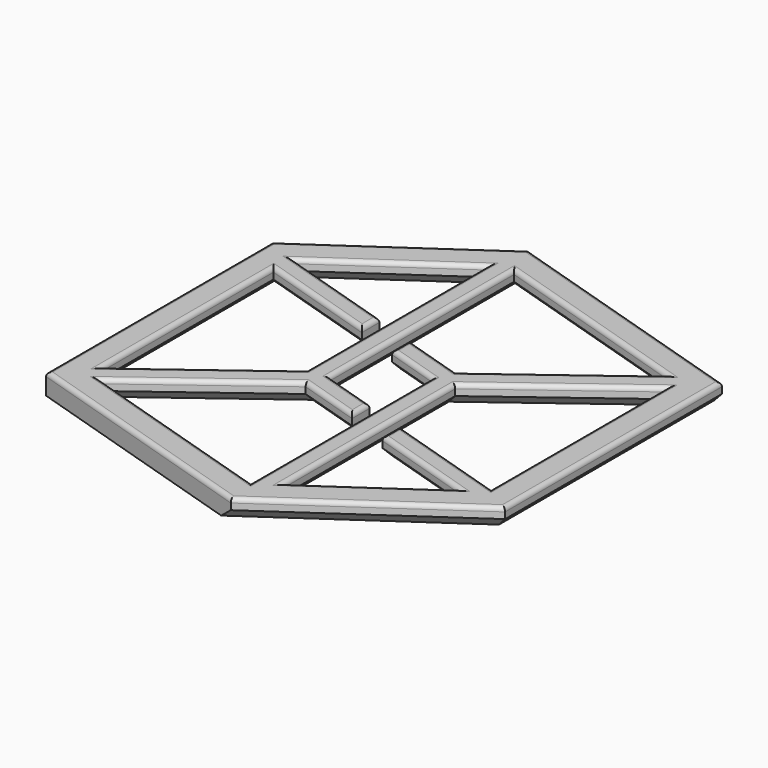
from build123d import *

# Parameters (mm, degrees)
F1_DEPTH = 2
F2_SIZE  = 0.99999
F3_R     = 0.4


# Not quite as in the source:
# - a fillet or chamfer is up to 0.001 mm smaller than in the source, because OpenCascade refuses the exact size
# - a feature names something its author has since deleted; it is built from what else it names


with BuildPart() as f1:
    # F0 (on Top) → F1 (new body)
    with BuildSketch(Plane.XY):
        Polygon((-13.8196714956, 16.8550248196), (-29.5628140081, 5.986613122), (-29.5628140081, -20.895469086), (-6.1378714726, -28.2046662626), (10.6815792442, -16.5932160853), (10.6815792442, 9.2099912209), align=None)
        Polygon((-5.5893215574, -24.5450593134), (-6.5893215574, -25.2354177783), (-25.6853743411, -19.2769478747), (-26.8628140101, -18.9095557801), (-26.8628140101, -17.6600457129), (-26.8628140101, 2.7856210558), (-26.8628140101, 4.569670104), (-26.5525036512, 4.783895487), (-14.6640113722, 12.9912167666), (-13.6640113722, 13.6815752315), (-13.3682214107, 13.8857763353), (-12.6640113722, 13.6660443117), (6.8041395773, 7.5914700096), (7.9815792463, 7.224077915), (7.9815792463, 5.9745678478), (7.9815792463, -14.864596124), (7.9815792463, -15.1762730673), (7.5702731242, -15.4602217303), (6.2023996294, -16.4045447763), (-4.5893215574, -23.8547008485), align=None, mode=Mode.SUBTRACT)
        Polygon((-26.8628140101, 4.569670104), (-26.8628140101, 2.7856210558), (-15.6640113722, -0.7086994318), (-15.6640113722, 1.3863999797), (-26.5525036512, 4.783895487), align=None)
        with BuildLine():
            Line((-13.6640113722, 13.6815752315), (-13.6640113722, -8.0212351043))
            ThreePointArc((-13.6640113722, -8.0212351043), (-13.5133605177, -8.0326480722), (-13.3661484098, -8.0666264642))
            Line((-13.3661484098, -8.0666264642), (-12.6640113722, -8.2857116571))
            Line((-12.6640113722, -8.2857116571), (-12.6640113722, 13.6660443117))
            Line((-12.6640113722, 13.6660443117), (-13.3682214107, 13.8857763353))
            Line((-13.3682214107, 13.8857763353), (-13.6640113722, 13.6815752315))
        make_face()
        with BuildLine():
            Line((-14.6640113722, 12.9912167666), (-14.6640113722, -8.5209081976))
            Line((-14.6640113722, -8.5209081976), (-14.2635929044, -8.2209214243))
            ThreePointArc((-14.2635929044, -8.2209214243), (-13.9799910551, -8.0724691479), (-13.6640113722, -8.0212351043))
            Line((-13.6640113722, -8.0212351043), (-13.6640113722, 13.6815752315))
            Line((-13.6640113722, 13.6815752315), (-14.6640113722, 12.9912167666))
        make_face()
        with BuildLine():
            Line((-6.5893215574, -3.6785358878), (-6.5893215574, -25.2354177783))
            Line((-6.5893215574, -25.2354177783), (-5.5893215574, -24.5450593134))
            Line((-5.5893215574, -24.5450593134), (-5.5893215574, -3.9430124406))
            ThreePointArc((-5.5893215574, -3.9430124406), (-5.739972412, -3.9315994727), (-5.8871845198, -3.8976210807))
            Line((-5.8871845198, -3.8976210807), (-6.5893215574, -3.6785358878))
        make_face()
        with BuildLine():
            Line((-5.5893215574, -3.9430124406), (-5.5893215574, -24.5450593134))
            Line((-5.5893215574, -24.5450593134), (-4.5893215574, -23.8547008485))
            Line((-4.5893215574, -23.8547008485), (-4.5893215574, -3.4433393473))
            Line((-4.5893215574, -3.4433393473), (-4.9897400253, -3.7433261206))
            ThreePointArc((-4.9897400253, -3.7433261206), (-5.2733418745, -3.891778397), (-5.5893215574, -3.9430124406))
        make_face()
        with BuildLine():
            ThreePointArc((-5.2914585951, -1.9884038006), (-5.0122521974, -2.1263172994), (-4.7890078775, -2.3434309085))
            Line((-4.7890078775, -2.3434309085), (7.9815792463, 7.224077915))
            Line((7.9815792463, 7.224077915), (6.8041395773, 7.5914700096))
            Line((6.8041395773, 7.5914700096), (-5.7796330622, -1.8360805481))
            Line((-5.7796330622, -1.8360805481), (-5.2914585951, -1.9884038006))
        make_face()
        with BuildLine():
            Line((-4.5893215574, -2.9430124406), (-4.5893215574, -3.4433393473))
            Line((-4.5893215574, -3.4433393473), (7.9815792463, 5.9745678478))
            Line((7.9815792463, 5.9745678478), (7.9815792463, 7.224077915))
            Line((7.9815792463, 7.224077915), (-4.7890078775, -2.3434309085))
            ThreePointArc((-4.7890078775, -2.3434309085), (-4.6405556011, -2.6270327577), (-4.5893215574, -2.9430124406))
        make_face()
        with BuildLine():
            Line((-26.8628140101, -18.9095557801), (-25.6853743411, -19.2769478747))
            Line((-25.6853743411, -19.2769478747), (-13.4736998674, -10.1281669968))
            Line((-13.4736998674, -10.1281669968), (-13.9618743346, -9.9758437443))
            ThreePointArc((-13.9618743346, -9.9758437443), (-14.2410807322, -9.8379302455), (-14.4643250521, -9.6208166364))
            Line((-14.4643250521, -9.6208166364), (-26.8628140101, -18.9095557801))
        make_face()
        with BuildLine():
            Line((-26.8628140101, -17.6600457129), (-26.8628140101, -18.9095557801))
            Line((-26.8628140101, -18.9095557801), (-14.4643250521, -9.6208166364))
            ThreePointArc((-14.4643250521, -9.6208166364), (-14.6127773286, -9.3372147872), (-14.6640113722, -9.0212351043))
            Line((-14.6640113722, -9.0212351043), (-14.6640113722, -8.5209081976))
            Line((-14.6640113722, -8.5209081976), (-26.8628140101, -17.6600457129))
        make_face()
        Polygon((-3.5893215574, -13.3492706494), (6.2023996294, -16.4045447763), (7.5702731242, -15.4602217303), (-3.5893215574, -11.9781351546), align=None)
        with BuildLine():
            Line((-11.6640113722, -2.0950994115), (-6.5893215574, -3.6785358878))
            Line((-6.5893215574, -3.6785358878), (-6.5893215574, -2.9430124406))
            ThreePointArc((-6.5893215574, -2.9430124406), (-6.4836317755, -2.4955649757), (-6.1889030896, -2.1426987607))
            Line((-6.1889030896, -2.1426987607), (-5.7796330622, -1.8360805481))
            Line((-5.7796330622, -1.8360805481), (-11.6640113722, 0))
            Line((-11.6640113722, 0), (-11.6640113722, -2.0950994115))
        make_face()
        with BuildLine():
            Line((-13.06442984, -9.8215487842), (-13.4736998674, -10.1281669968))
            Line((-13.4736998674, -10.1281669968), (-7.5893215574, -11.9642475449))
            Line((-7.5893215574, -11.9642475449), (-7.5893215574, -9.8691481334))
            Line((-7.5893215574, -9.8691481334), (-12.6640113722, -8.2857116571))
            Line((-12.6640113722, -8.2857116571), (-12.6640113722, -9.0212351043))
            ThreePointArc((-12.6640113722, -9.0212351043), (-12.7697011542, -9.4686825693), (-13.06442984, -9.8215487842))
        make_face()
        Polygon((-3.5893215574, -11.9781351546), (7.5702731242, -15.4602217303), (7.9815792463, -15.1762730673), (7.9815792463, -14.864596124), (-3.5893215574, -11.2541712379), align=None)
        with BuildLine():
            ThreePointArc((-5.8871845198, -3.8976210807), (-5.739972412, -3.9315994727), (-5.5893215574, -3.9430124406))
            Line((-5.5893215574, -3.9430124406), (-5.5893215574, -2.9430124406))
            Line((-5.5893215574, -2.9430124406), (-4.7890078775, -2.3434309085))
            ThreePointArc((-4.7890078775, -2.3434309085), (-5.0122521974, -2.1263172994), (-5.2914585951, -1.9884038006))
            ThreePointArc((-5.2914585951, -1.9884038006), (-5.7587625723, -1.9574721104), (-6.1889030896, -2.1426987607))
            ThreePointArc((-6.1889030896, -2.1426987607), (-6.4836317755, -2.4955649757), (-6.5893215574, -2.9430124406))
            ThreePointArc((-6.5893215574, -2.9430124406), (-6.3948843925, -3.535522794), (-5.8871845198, -3.8976210807))
        make_face()
        with BuildLine():
            Line((-13.6640113722, -9.0212351043), (-14.4643250521, -9.6208166364))
            ThreePointArc((-14.4643250521, -9.6208166364), (-14.2410807322, -9.8379302455), (-13.9618743346, -9.9758437443))
            ThreePointArc((-13.9618743346, -9.9758437443), (-13.4945703573, -10.0067754345), (-13.06442984, -9.8215487842))
            ThreePointArc((-13.06442984, -9.8215487842), (-12.7697011542, -9.4686825693), (-12.6640113722, -9.0212351043))
            ThreePointArc((-12.6640113722, -9.0212351043), (-12.8584485372, -8.4287247509), (-13.3661484098, -8.0666264642))
            ThreePointArc((-13.3661484098, -8.0666264642), (-13.5133605177, -8.0326480722), (-13.6640113722, -8.0212351043))
            Line((-13.6640113722, -8.0212351043), (-13.6640113722, -9.0212351043))
        make_face()
        with BuildLine():
            Line((-5.5893215574, -2.9430124406), (-5.5893215574, -3.9430124406))
            ThreePointArc((-5.5893215574, -3.9430124406), (-5.2733418745, -3.891778397), (-4.9897400253, -3.7433261206))
            ThreePointArc((-4.9897400253, -3.7433261206), (-4.6950113394, -3.3904599056), (-4.5893215574, -2.9430124406))
            ThreePointArc((-4.5893215574, -2.9430124406), (-4.6405556011, -2.6270327577), (-4.7890078775, -2.3434309085))
            Line((-4.7890078775, -2.3434309085), (-5.5893215574, -2.9430124406))
        make_face()
        with BuildLine():
            ThreePointArc((-14.6640113722, -9.0212351043), (-14.6127773286, -9.3372147872), (-14.4643250521, -9.6208166364))
            Line((-14.4643250521, -9.6208166364), (-13.6640113722, -9.0212351043))
            Line((-13.6640113722, -9.0212351043), (-13.6640113722, -8.0212351043))
            ThreePointArc((-13.6640113722, -8.0212351043), (-13.9799910551, -8.0724691479), (-14.2635929044, -8.2209214243))
            ThreePointArc((-14.2635929044, -8.2209214243), (-14.5583215902, -8.5737876393), (-14.6640113722, -9.0212351043))
        make_face()
        with BuildLine():
            Line((-6.5893215574, -2.9430124406), (-6.5893215574, -3.6785358878))
            Line((-6.5893215574, -3.6785358878), (-5.8871845198, -3.8976210807))
            ThreePointArc((-5.8871845198, -3.8976210807), (-6.3948843925, -3.535522794), (-6.5893215574, -2.9430124406))
        make_face()
        with BuildLine():
            ThreePointArc((-13.3661484098, -8.0666264642), (-12.8584485372, -8.4287247509), (-12.6640113722, -9.0212351043))
            Line((-12.6640113722, -9.0212351043), (-12.6640113722, -8.2857116571))
            Line((-12.6640113722, -8.2857116571), (-13.3661484098, -8.0666264642))
        make_face()
        with BuildLine():
            Line((-13.9618743346, -9.9758437443), (-13.4736998674, -10.1281669968))
            Line((-13.4736998674, -10.1281669968), (-13.06442984, -9.8215487842))
            ThreePointArc((-13.06442984, -9.8215487842), (-13.4945703573, -10.0067754345), (-13.9618743346, -9.9758437443))
        make_face()
        with BuildLine():
            Line((-5.7796330622, -1.8360805481), (-6.1889030896, -2.1426987607))
            ThreePointArc((-6.1889030896, -2.1426987607), (-5.7587625723, -1.9574721104), (-5.2914585951, -1.9884038006))
            Line((-5.2914585951, -1.9884038006), (-5.7796330622, -1.8360805481))
        make_face()
        with BuildLine():
            Line((-4.9897400253, -3.7433261206), (-4.5893215574, -3.4433393473))
            Line((-4.5893215574, -3.4433393473), (-4.5893215574, -2.9430124406))
            ThreePointArc((-4.5893215574, -2.9430124406), (-4.6950113394, -3.3904599056), (-4.9897400253, -3.7433261206))
        make_face()
        with BuildLine():
            Line((-14.2635929044, -8.2209214243), (-14.6640113722, -8.5209081976))
            Line((-14.6640113722, -8.5209081976), (-14.6640113722, -9.0212351043))
            ThreePointArc((-14.6640113722, -9.0212351043), (-14.5583215902, -8.5737876393), (-14.2635929044, -8.2209214243))
        make_face()
    extrude(amount=F1_DEPTH)

    # F2 (size 1 in the source; OpenCascade refuses exactly that, so slightly less here)
    f2_edges = [f1.edges().sort_by_distance(p)[0] for p in [
        (-6.589322, -14.456977, 0),
        (-12.664011, 2.690166, 0),
        (-20.608258, 8.887556, 0),
        (-26.862814, -7.437212, 0),
        (-21.263413, 1.038461, 0),
        (-19.579537, -14.702557, 0),
        (1.306539, -14.876908, 0),
        (-10.531511, -11.046207, 0),
        (-9.126666, -2.886818, 0),
        (-4.589322, -13.64902, 0),
        (1.696129, 1.265614, 0),
        (10.681579, -3.691612, 0),
        (-2.929936, 10.628757, 0),
        (2.271854, -22.398941, 0),
        (-16.137348, -22.256183, 0),
    ]]
    chamfer(f2_edges, length=F2_SIZE)

    # F3
    f3_edges = [f1.edges().sort_by_distance(p)[0] for p in [
        (-17.850343, -24.550068, 2),
        (2.271854, -22.398941, 2),
        (10.681579, -3.691612, 2),
        (-1.569046, 13.032508, 2),
        (-21.691243, 11.420819, 2),
        (-29.562814, -7.454428, 2),
        (7.981579, -4.445014, 2),
        (0.806539, -20.129623, 2),
        (-16.137348, -22.256183, 2),
        (-26.862814, -7.437212, 2),
        (-21.263413, 1.038461, 2),
        (-21.108258, 3.085148, 2),
        (-14.664011, 2.235154, 2),
        (-12.664011, 2.690166, 2),
        (1.696129, 1.265614, 2),
        (0.512253, 2.877695, 2),
        (-4.589322, -13.64902, 2),
        (2.196129, -13.059384, 2),
        (-3.589322, -12.301721, 2),
        (1.306539, -14.876908, 2),
        (-20.763413, -13.090477, 2),
        (-15.664011, 0.33885, 2),
        (-20.608258, 8.887556, 2),
        (-8.721822, -0.91804, 2),
        (-11.664011, -1.04755, 2),
        (-9.126666, -2.886818, 2),
        (-6.589322, -14.456977, 2),
        (-19.579537, -14.702557, 2),
        (-10.531511, -11.046207, 2),
        (-7.589322, -10.916698, 2),
        (-10.126666, -9.07743, 2),
        (-2.929936, 10.628757, 2),
    ]]
    fillet(f3_edges, radius=F3_R)


solid = f1.part
